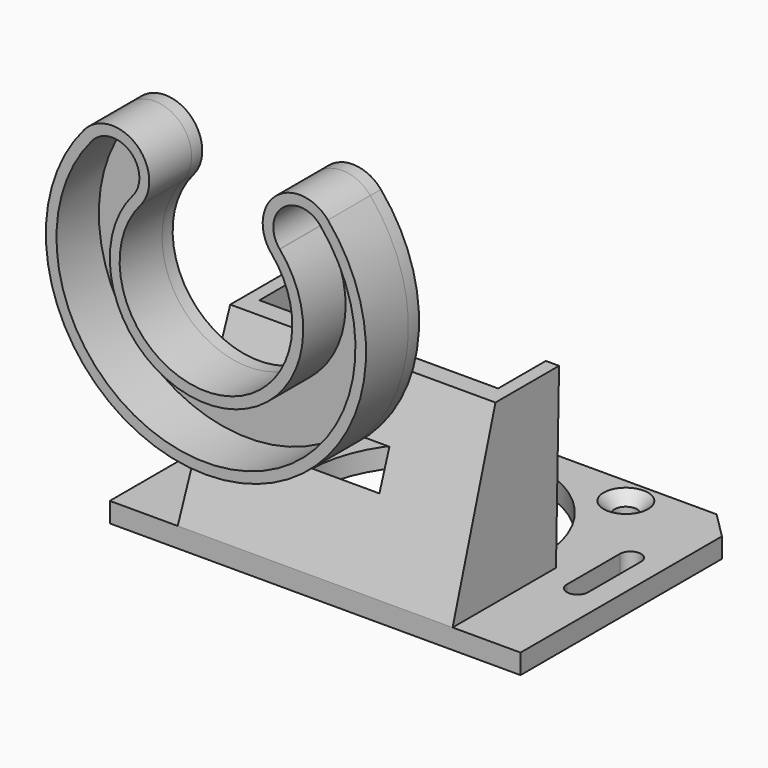
from build123d import *
from build123d import SkipClean  # not in build123d's __all__

# Parameters (mm, degrees)
F0_W           = 10
F0_H           = 12
F0_W_2         = 9.9836443961
F1_DEPTH       = 3
F2_D           = 3.4
F2_CSINK_D     = 6.72
F2_CSINK_ANGLE = 90
F3_SIZE        = 4
F9_W           = 24
F9_H           = 5
F10_DEPTH      = 15
F15_DEPTH      = 8
F17_DEPTH      = 2


# Not quite as in the source:
# - a feature names something its author has since deleted; it is built from what else it names


with BuildPart() as f1:
    # F0 (on Top) → F1 (new body)
    with BuildSketch(Plane.XY):
        with Locations((-26, -15)):
            Rectangle(F0_W, F0_H)
        with Locations((26.008177802, -15)):
            Rectangle(F0_W_2, F0_H)
        Polygon((31, 21), (-31, 21), (-31, -9), (-21, -9), (-21, -21), (21.0163556039, -21), (21.0163556039, -9), (31, -9), align=None)
        with BuildLine():
            ThreePointArc((-24.4, -4), (-26, -5.6), (-27.6, -4))
            Line((-27.6, -4), (-27.6, 6))
            ThreePointArc((-27.6, 6), (-26, 7.6), (-24.4, 6))
            Line((-24.4, 6), (-24.4, -4))
        make_face(mode=Mode.SUBTRACT)
        with BuildLine():
            ThreePointArc((-17.5, 0), (0, 17.5), (17.5, 0))
            Line((17.5, 0), (17.5, -5.5))
            ThreePointArc((17.5, -5.5), (13.9852813742, -13.9852813742), (5.5, -17.5))
            Line((5.5, -17.5), (-15.5, -17.5))
            ThreePointArc((-15.5, -17.5), (-16.9142135624, -16.9142135624), (-17.5, -15.5))
            Line((-17.5, -15.5), (-17.5, 0))
        make_face(mode=Mode.SUBTRACT)
        with BuildLine():
            ThreePointArc((27.6, -4), (26, -5.6), (24.4, -4))
            Line((24.4, -4), (24.4, 6))
            ThreePointArc((24.4, 6), (26, 7.6), (27.6, 6))
            Line((27.6, 6), (27.6, -4))
        make_face(mode=Mode.SUBTRACT)
    extrude(amount=-F1_DEPTH)

    # F2 (through all)
    with Locations(Plane.XY):
        with Locations((-16.5, 17), (16.5, 17)):
            CounterSinkHole(F2_D / 2, F2_CSINK_D / 2, counter_sink_angle=F2_CSINK_ANGLE)

    # F3
    f3_edges = [f1.edges().sort_by_distance(p)[0] for p in [
        (31, 21, -1.5),
        (-31, 21, -1.5),
    ]]
    chamfer(f3_edges, length=F3_SIZE)

    # F4 (on face) → F7 section 0
    with BuildSketch(Plane.XY):
        Polygon((-18.75, -1.5), (-20.75, -1.5), (-20.75, -21), (20.75, -21), (20.75, -1.5), (18.75, -1.5), (18.75, -18), (-18.75, -18), align=None)
    # F6 (on offset) → F7 section 1
    with BuildSketch(Plane.XY.offset(26)):
        Polygon((-20.0163556039, 0), (-20.0163556039, -12), (20.0163556039, -12), (20.0163556039, 0), (18.0163556039, 0), (18.0163556039, -9), (-18.0163556039, -9), (-18.0163556039, 0), align=None)
    loft()

    # F9 (on offset) → F10 (cut)
    with BuildSketch(Plane.XY.offset(2)):
        with Locations((-5.5, -14.5)):
            Rectangle(F9_W, F9_H)
    extrude(amount=F10_DEPTH, mode=Mode.SUBTRACT)


with BuildPart() as f15:
    # F13 (on offset) → F15 (new body)
    with BuildSketch(Plane.XZ.offset(31)):
        with BuildLine():
            ThreePointArc((-18.3830856085, 47.4395647135), (-19.0105652692, 55.3219802644), (-26.8929808201, 54.6945006036))
            ThreePointArc((-26.8929808201, 54.6945006036), (-8.4836443961, 14.8667804257), (9.9256920279, 54.6945006036))
            ThreePointArc((9.9256920279, 54.6945006036), (2.0432764771, 55.3219802644), (1.4157968163, 47.4395647135))
            ThreePointArc((1.4157968163, 47.4395647135), (-8.4836443961, 25.9331770523), (-18.3830856085, 47.4395647135))
        make_face()
        with BuildLine():
            ThreePointArc((8.7375378537, 53.6218026281), (-8.5063834027, 16.4667918811), (-25.6753981826, 53.6564756038))
            ThreePointArc((-25.6753981826, 53.6564756038), (-19.959761381, 54.1114688502), (-19.5047681345, 48.3958320486))
            ThreePointArc((-19.5047681345, 48.3958320486), (-8.3719987512, 24.316495823), (2.666209427, 48.439326242))
            ThreePointArc((2.666209427, 48.439326242), (2.6497503397, 48.4584205612), (2.6332583079, 48.4774864329))
            ThreePointArc((2.6332583079, 48.4774864329), (3.0985445837, 54.1192219614), (8.7375378537, 53.6218026281))
        make_face(mode=Mode.SUBTRACT)
    extrude(amount=-F15_DEPTH)

    # F16 (on face) → F17 (join)
    with BuildSketch(Plane(origin=(0, -23, 0), x_dir=(-1, 0, 0), z_dir=(0, 1, 0))):
        with BuildLine():
            ThreePointArc((26.8929808201, 54.6945006036), (19.0105652692, 55.3219802644), (18.3830856085, 47.4395647135))
            ThreePointArc((18.3830856085, 47.4395647135), (8.4836443961, 25.9331770523), (-1.4157968163, 47.4395647135))
            ThreePointArc((-1.4157968163, 47.4395647135), (-2.0432764771, 55.3219802644), (-9.9256920279, 54.6945006036))
            ThreePointArc((-9.9256920279, 54.6945006036), (8.4836443961, 14.8667804257), (26.8929808201, 54.6945006036))
        make_face()
    with SkipClean():  # cleaning this boolean's faces spoils the solid; the shape is the same uncleaned
        extrude(amount=F17_DEPTH)


solid = Compound([f1.part, f15.part])
